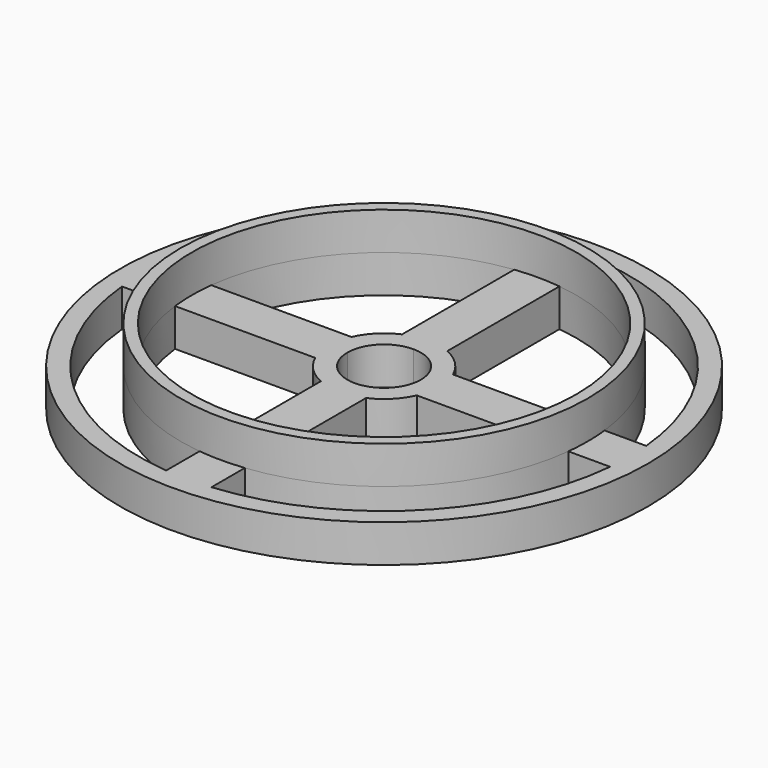
from build123d import *

# Parameters (mm, degrees)
F0_R     = 35
F1_DEPTH = 5
F2_R     = 27
F2_R_2   = 25.5
F3_DEPTH = 5


with BuildPart() as f1:
    # F0 (on Top) → F1 (new body)
    with BuildSketch(Plane.XY):
        Circle(F0_R)
        with BuildLine():
            ThreePointArc((3, 32.3612422506), (22.9809703886, 22.9809703886), (32.3612422506, 3))
            ThreePointArc((32.3612422506, 3), (32.4652920297, 1.5016036189), (32.5, 0))
            ThreePointArc((32.5, 0), (32.4652920297, -1.5016036189), (32.3612422506, -3))
            ThreePointArc((32.3612422506, -3), (22.9809703886, -22.9809703886), (3, -32.3612422506))
            ThreePointArc((3, -32.3612422506), (0, -32.5), (-3, -32.3612422506))
            ThreePointArc((-3, -32.3612422506), (-22.9809703886, -22.9809703886), (-32.3612422506, -3))
            ThreePointArc((-32.3612422506, -3), (-32.5, 0), (-32.3612422506, 3))
            ThreePointArc((-32.3612422506, 3), (-22.9809703886, 22.9809703886), (-3, 32.3612422506))
            ThreePointArc((-3, 32.3612422506), (0, 32.5), (3, 32.3612422506))
        make_face(mode=Mode.SUBTRACT)
        with BuildLine():
            ThreePointArc((-6.7372564891, -3), (-7.2138024511, -1.5335185674), (-7.375, 0))
            ThreePointArc((-7.375, 0), (-7.2138024511, 1.5335185674), (-6.7372564891, 3))
            Line((-6.7372564891, 3), (-23.8117617996, 3))
            ThreePointArc((-23.8117617996, 3), (-24, 0), (-23.8117617996, -3))
            Line((-23.8117617996, -3), (-6.7372564891, -3))
        make_face()
        with BuildLine():
            ThreePointArc((-4.875, 0), (-3.4471455583, 3.4471455583), (0, 4.875))
            Line((0, 4.875), (0, 7.375))
            ThreePointArc((0, 7.375), (-1.5335185674, 7.2138024511), (-3, 6.7372564891))
            ThreePointArc((-3, 6.7372564891), (-5.2149125113, 5.2149125113), (-6.7372564891, 3))
            ThreePointArc((-6.7372564891, 3), (-7.2138024511, 1.5335185674), (-7.375, 0))
            Line((-7.375, 0), (-4.875, 0))
        make_face()
        with BuildLine():
            Line((0, -7.375), (0, -4.875))
            ThreePointArc((0, -4.875), (-3.4471455583, -3.4471455583), (-4.875, 0))
            Line((-4.875, 0), (-7.375, 0))
            ThreePointArc((-7.375, 0), (-7.2138024511, -1.5335185674), (-6.7372564891, -3))
            ThreePointArc((-6.7372564891, -3), (-5.2149125113, -5.2149125113), (-3, -6.7372564891))
            ThreePointArc((-3, -6.7372564891), (-1.5335185674, -7.2138024511), (0, -7.375))
        make_face()
        with BuildLine():
            Line((7.375, 0), (4.875, 0))
            ThreePointArc((4.875, 0), (3.4471455583, -3.4471455583), (0, -4.875))
            Line((0, -4.875), (0, -7.375))
            ThreePointArc((0, -7.375), (1.5335185674, -7.2138024511), (3, -6.7372564891))
            ThreePointArc((3, -6.7372564891), (5.2149125113, -5.2149125113), (6.7372564891, -3))
            ThreePointArc((6.7372564891, -3), (7.2138024511, -1.5335185674), (7.375, 0))
        make_face()
        with BuildLine():
            ThreePointArc((0, 4.875), (3.4471455583, 3.4471455583), (4.875, 0))
            Line((4.875, 0), (7.375, 0))
            ThreePointArc((7.375, 0), (7.2138024511, 1.5335185674), (6.7372564891, 3))
            ThreePointArc((6.7372564891, 3), (5.2149125113, 5.2149125113), (3, 6.7372564891))
            ThreePointArc((3, 6.7372564891), (1.5335185674, 7.2138024511), (0, 7.375))
            Line((0, 7.375), (0, 4.875))
        make_face()
        with BuildLine():
            ThreePointArc((-3, 6.7372564891), (-1.5335185674, 7.2138024511), (0, 7.375))
            ThreePointArc((0, 7.375), (1.5335185674, 7.2138024511), (3, 6.7372564891))
            Line((3, 6.7372564891), (3, 23.8117617996))
            ThreePointArc((3, 23.8117617996), (0, 24), (-3, 23.8117617996))
            Line((-3, 23.8117617996), (-3, 6.7372564891))
        make_face()
        with BuildLine():
            ThreePointArc((6.7372564891, 3), (7.2138024511, 1.5335185674), (7.375, 0))
            ThreePointArc((7.375, 0), (7.2138024511, -1.5335185674), (6.7372564891, -3))
            Line((6.7372564891, -3), (23.8117617996, -3))
            ThreePointArc((23.8117617996, -3), (23.9528942217, -1.502949901), (24, 0))
            ThreePointArc((24, 0), (23.9528942217, 1.502949901), (23.8117617996, 3))
            Line((23.8117617996, 3), (6.7372564891, 3))
        make_face()
        with BuildLine():
            ThreePointArc((3, -6.7372564891), (1.5335185674, -7.2138024511), (0, -7.375))
            ThreePointArc((0, -7.375), (-1.5335185674, -7.2138024511), (-3, -6.7372564891))
            Line((-3, -6.7372564891), (-3, -23.8117617996))
            ThreePointArc((-3, -23.8117617996), (0, -24), (3, -23.8117617996))
            Line((3, -23.8117617996), (3, -6.7372564891))
        make_face()
        with BuildLine():
            ThreePointArc((-3, 23.8117617996), (0, 24), (3, 23.8117617996))
            Line((3, 23.8117617996), (3, 25.3229145242))
            ThreePointArc((3, 25.3229145242), (0, 25.5), (-3, 25.3229145242))
            Line((-3, 25.3229145242), (-3, 23.8117617996))
        make_face()
        with BuildLine():
            ThreePointArc((-3, 25.3229145242), (0, 25.5), (3, 25.3229145242))
            Line((3, 25.3229145242), (3, 26.83281573))
            ThreePointArc((3, 26.83281573), (0, 27), (-3, 26.83281573))
            Line((-3, 26.83281573), (-3, 25.3229145242))
        make_face()
        with BuildLine():
            ThreePointArc((-3, 26.83281573), (0, 27), (3, 26.83281573))
            Line((3, 26.83281573), (3, 32.3612422506))
            ThreePointArc((3, 32.3612422506), (0, 32.5), (-3, 32.3612422506))
            Line((-3, 32.3612422506), (-3, 26.83281573))
        make_face()
        with BuildLine():
            Line((25.3229145242, 3), (23.8117617996, 3))
            ThreePointArc((23.8117617996, 3), (23.9528942217, 1.502949901), (24, 0))
            ThreePointArc((24, 0), (23.9528942217, -1.502949901), (23.8117617996, -3))
            Line((23.8117617996, -3), (25.3229145242, -3))
            ThreePointArc((25.3229145242, -3), (25.4556901337, -1.5026109997), (25.5, 0))
            ThreePointArc((25.5, 0), (25.4556901337, 1.5026109997), (25.3229145242, 3))
        make_face()
        with BuildLine():
            Line((26.83281573, 3), (25.3229145242, 3))
            ThreePointArc((25.3229145242, 3), (25.4556901337, 1.5026109997), (25.5, 0))
            ThreePointArc((25.5, 0), (25.4556901337, -1.5026109997), (25.3229145242, -3))
            Line((25.3229145242, -3), (26.83281573, -3))
            ThreePointArc((26.83281573, -3), (26.9581715321, -1.5023274094), (27, 0))
            ThreePointArc((27, 0), (26.9581715321, 1.5023274094), (26.83281573, 3))
        make_face()
        with BuildLine():
            Line((32.3612422506, 3), (26.83281573, 3))
            ThreePointArc((26.83281573, 3), (26.9581715321, 1.5023274094), (27, 0))
            ThreePointArc((27, 0), (26.9581715321, -1.5023274094), (26.83281573, -3))
            Line((26.83281573, -3), (32.3612422506, -3))
            ThreePointArc((32.3612422506, -3), (32.4652920297, -1.5016036189), (32.5, 0))
            ThreePointArc((32.5, 0), (32.4652920297, 1.5016036189), (32.3612422506, 3))
        make_face()
        with BuildLine():
            ThreePointArc((-23.8117617996, -3), (-24, 0), (-23.8117617996, 3))
            Line((-23.8117617996, 3), (-25.3229145242, 3))
            ThreePointArc((-25.3229145242, 3), (-25.5, 0), (-25.3229145242, -3))
            Line((-25.3229145242, -3), (-23.8117617996, -3))
        make_face()
        with BuildLine():
            ThreePointArc((-25.3229145242, -3), (-25.5, 0), (-25.3229145242, 3))
            Line((-25.3229145242, 3), (-26.83281573, 3))
            ThreePointArc((-26.83281573, 3), (-27, 0), (-26.83281573, -3))
            Line((-26.83281573, -3), (-25.3229145242, -3))
        make_face()
        with BuildLine():
            ThreePointArc((-26.83281573, -3), (-27, 0), (-26.83281573, 3))
            Line((-26.83281573, 3), (-32.3612422506, 3))
            ThreePointArc((-32.3612422506, 3), (-32.5, 0), (-32.3612422506, -3))
            Line((-32.3612422506, -3), (-26.83281573, -3))
        make_face()
        with BuildLine():
            ThreePointArc((3, -23.8117617996), (0, -24), (-3, -23.8117617996))
            Line((-3, -23.8117617996), (-3, -25.3229145242))
            ThreePointArc((-3, -25.3229145242), (0, -25.5), (3, -25.3229145242))
            Line((3, -25.3229145242), (3, -23.8117617996))
        make_face()
        with BuildLine():
            ThreePointArc((3, -25.3229145242), (0, -25.5), (-3, -25.3229145242))
            Line((-3, -25.3229145242), (-3, -26.83281573))
            ThreePointArc((-3, -26.83281573), (0, -27), (3, -26.83281573))
            Line((3, -26.83281573), (3, -25.3229145242))
        make_face()
        with BuildLine():
            ThreePointArc((3, -26.83281573), (0, -27), (-3, -26.83281573))
            Line((-3, -26.83281573), (-3, -32.3612422506))
            ThreePointArc((-3, -32.3612422506), (0, -32.5), (3, -32.3612422506))
            Line((3, -32.3612422506), (3, -26.83281573))
        make_face()
        with BuildLine():
            ThreePointArc((-25.3229145242, 3), (-18.0312229203, 18.0312229203), (-3, 25.3229145242))
            Line((-3, 25.3229145242), (-3, 26.83281573))
            ThreePointArc((-3, 26.83281573), (-19.091883092, 19.091883092), (-26.83281573, 3))
            Line((-26.83281573, 3), (-25.3229145242, 3))
        make_face()
        with BuildLine():
            ThreePointArc((3, 25.3229145242), (18.0312229203, 18.0312229203), (25.3229145242, 3))
            Line((25.3229145242, 3), (26.83281573, 3))
            ThreePointArc((26.83281573, 3), (19.091883092, 19.091883092), (3, 26.83281573))
            Line((3, 26.83281573), (3, 25.3229145242))
        make_face()
        with BuildLine():
            Line((26.83281573, -3), (25.3229145242, -3))
            ThreePointArc((25.3229145242, -3), (18.0312229203, -18.0312229203), (3, -25.3229145242))
            Line((3, -25.3229145242), (3, -26.83281573))
            ThreePointArc((3, -26.83281573), (19.091883092, -19.091883092), (26.83281573, -3))
        make_face()
        with BuildLine():
            Line((-3, -26.83281573), (-3, -25.3229145242))
            ThreePointArc((-3, -25.3229145242), (-18.0312229203, -18.0312229203), (-25.3229145242, -3))
            Line((-25.3229145242, -3), (-26.83281573, -3))
            ThreePointArc((-26.83281573, -3), (-19.091883092, -19.091883092), (-3, -26.83281573))
        make_face()
    extrude(amount=F1_DEPTH)

    # F2 (on face) → F3 (join)
    with BuildSketch(Plane.XY.offset(5)):
        Circle(F2_R)
        Circle(F2_R_2, mode=Mode.SUBTRACT)
    extrude(amount=F3_DEPTH)


solid = f1.part
